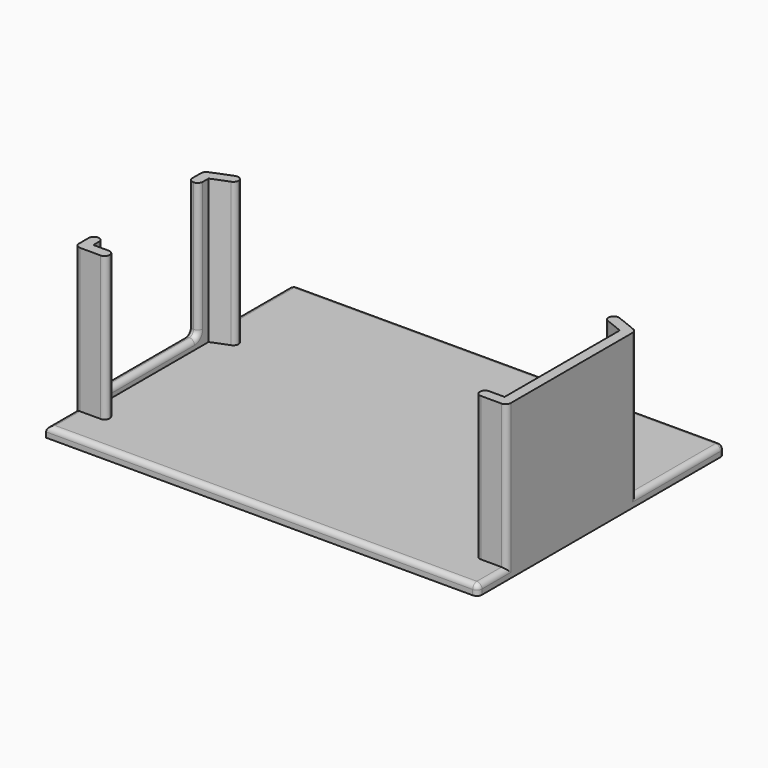
from build123d import *

# Parameters (mm, degrees)
F0_W     = 72
F0_H     = 2
F1_DEPTH = 2
F2_DEPTH = 30
F3_W     = 23.2293857262
F3_H     = 26.1833476555
F4_DEPTH = 2
F5_R     = 0.99999


# Not quite as in the source:
# - a fillet or chamfer is up to 0.001 mm smaller than in the source, because OpenCascade refuses the exact size


with BuildPart() as f1:
    # F0 (on Top) → F1 (new body)
    with BuildSketch(Plane.XY):
        with BuildLine():
            ThreePointArc((-36, 15.5704873412), (0, 22), (36, 15.5704873412))
            Line((36, 15.5704873412), (36, 17.6995486449))
            ThreePointArc((36, 17.6995486449), (0, 24), (-36, 17.6995486449))
            Line((-36, 17.6995486449), (-36, 15.5704873412))
        make_face()
        with BuildLine():
            Line((-40, 14), (40, 14))
            ThreePointArc((40, 14), (38.0081123923, 14.8059057722), (36, 15.5704873412))
            ThreePointArc((36, 15.5704873412), (0, 22), (-36, 15.5704873412))
            ThreePointArc((-36, 15.5704873412), (-38.0081123923, 14.8059057722), (-40, 14))
        make_face()
        Polygon((36, -14), (40, -14), (40, 14), (-40, 14), (-40, -14), (-36, -14), align=None)
        with Locations((0, -15)):
            Rectangle(F0_W, F0_H)
        with BuildLine():
            ThreePointArc((-36, 17.6995486449), (0, 24), (36, 17.6995486449))
            ThreePointArc((36, 17.6995486449), (39.0180800363, 16.5575437512), (42, 15.3242004848))
            Line((42, 15.3242004848), (42, 37))
            Line((42, 37), (-42, 37))
            Line((-42, 37), (-42, 15.3242004848))
            ThreePointArc((-42, 15.3242004848), (-39.0180800363, 16.5575437512), (-36, 17.6995486449))
        make_face()
        Polygon((42, -16), (36, -16), (-36, -16), (-42, -16), (-42, -23), (42, -23), align=None)
    extrude(amount=F1_DEPTH)

    # F0 (on Top) → F2 (join)
    with BuildSketch(Plane.XY):
        with BuildLine():
            Line((-36, -16), (-36, -14))
            Line((-36, -14), (-40, -14))
            Line((-40, -14), (-40, 14))
            ThreePointArc((-40, 14), (-38.0081123923, 14.8059057722), (-36, 15.5704873412))
            Line((-36, 15.5704873412), (-36, 17.6995486449))
            ThreePointArc((-36, 17.6995486449), (-39.0180800363, 16.5575437512), (-42, 15.3242004848))
            Line((-42, 15.3242004848), (-42, -16))
            Line((-42, -16), (-36, -16))
        make_face()
        with BuildLine():
            Line((40, 14), (40, -14))
            Line((40, -14), (36, -14))
            Line((36, -14), (36, -16))
            Line((36, -16), (42, -16))
            Line((42, -16), (42, 15.3242004848))
            ThreePointArc((42, 15.3242004848), (39.0180800363, 16.5575437512), (36, 17.6995486449))
            Line((36, 17.6995486449), (36, 15.5704873412))
            ThreePointArc((36, 15.5704873412), (38.0081123923, 14.8059057722), (40, 14))
        make_face()
    extrude(amount=F2_DEPTH)

    # F3 (on face) → F4 (cut, through all)
    with BuildSketch(Plane(origin=(-42, 0, 0), x_dir=(0, -1, 0), z_dir=(-1, 0, 0))):
        with Locations((0.0190031715, 16.9083261723)):
            Rectangle(F3_W, F3_H)
    extrude(amount=-F4_DEPTH, mode=Mode.SUBTRACT)

    # F5 (radius 1 in the source; OpenCascade refuses exactly that, so slightly less here)
    f5_edges = [f1.edges().sort_by_distance(p)[0] for p in [
        (0, -23, 2),
        (42, -23, 1),
        (42, -19.5, 2),
        (-42, -19.5, 2),
        (-42, 26.1621, 2),
        (0, 37, 2),
        (-42, 37, 1),
        (42, 26.1621, 2),
        (42, 37, 1),
        (42, 15.3242, 16),
        (42, -16, 16),
        (36, 17.699549, 16),
        (36, 15.570487, 16),
        (36, -16, 16),
        (36, -14, 16),
        (-42, 15.3242, 16),
        (-36, 17.699549, 16),
        (-42, 11.59569, 16.908326),
        (-42, -11.633696, 16.908326),
        (-42, -16, 16),
        (-36, -16, 16),
        (-36, -14, 16),
        (-36, 15.570487, 16),
        (-40, -11.633696, 16.908326),
        (-40, 11.59569, 16.908326),
        (-42, -0.019003, 3.816652),
        (-40, -0.019003, 3.816652),
        (-41, -11.633696, 3.816652),
        (-41, 11.59569, 3.816652),
    ]]
    fillet(f5_edges, radius=F5_R)


solid = f1.part
